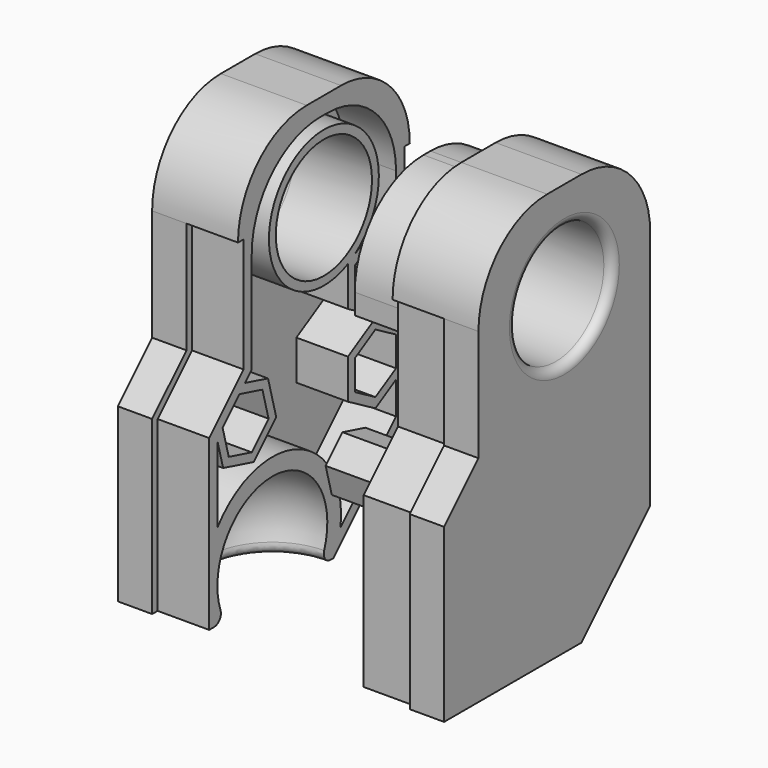
from build123d import *

# Parameters (mm, degrees)
F1_DEPTH  = 5
F4_R      = 3.5
F5_DEPTH  = 25
F7_DEPTH  = 3
F9_R      = 5
F11_DEPTH = 6
F13_DEPTH = 6
F14_R     = 0.5
F14_2_R   = 0.5
F16_DEPTH = 3
F18_DEPTH = 3


with BuildPart() as f1:
    # F0 (on Right) → F1 (new body)
    with BuildSketch(Plane.YZ):
        Polygon((0, 10), (0, 0), (10, 0), (15, 5), (15, 20), (15, 24), (2.5, 24), (2.5, 20), (2.5, 12.5), align=None)
    extrude(amount=F1_DEPTH)

    # F2 (on face) → F3 (revolve, cut)
    with BuildSketch(Plane.YZ.offset(5)):
        with BuildLine():
            Line((5, -2), (5, 6))
            ThreePointArc((5, 6), (1, 2), (5, -2))
        make_face()
    revolve(axis=Axis((5, 5, 2), (0, 0, -1)), mode=Mode.SUBTRACT)

    # F4 (on face) → F5 (cut)
    with BuildSketch(Plane.YZ.offset(5)):
        with Locations((8.75, 18.25)):
            Circle(F4_R)
    extrude(amount=-F5_DEPTH, mode=Mode.SUBTRACT)

    # F6 (on face) → F7 (cut)
    with BuildSketch(Plane.YZ.offset(5)):
        with BuildLine():
            Line((1.4182789124, 7.8827450064), (1, 9.4437831591))
            Line((1, 9.4437831591), (1, 5))
            ThreePointArc((1, 5), (6.8750834794, 6.6350902845), (9.9607833148, 1.3749968772))
            Line((9.9607833148, 1.3749968772), (14, 5.4142135624))
            Line((14, 5.4142135624), (14, 7.3028310874))
            Line((14, 7.3028310874), (12.5, 6.4368056836))
            Line((12.5, 6.4368056836), (10.5, 7.591506222))
            Line((10.5, 7.591506222), (10.5, 9.9009072988))
            Line((10.5, 9.9009072988), (12.5, 11.0556078372))
            Line((12.5, 11.0556078372), (14, 10.1895824334))
            Line((14, 10.1895824334), (14, 12.056624327))
            Line((14, 12.056624327), (12.5, 11.1905989232))
            Line((12.5, 11.1905989232), (10.5, 12.3452994616))
            Line((10.5, 12.3452994616), (10.5, 14.6531263575))
            ThreePointArc((10.5, 14.6531263575), (5.3588350084, 20.3713203436), (12.75, 18.25))
            ThreePointArc((12.75, 18.25), (12.2870669156, 16.3820712982), (11.0054211826, 14.9465055942))
            Line((11.0054211826, 14.9465055942), (12.5, 15.8094010768))
            Line((12.5, 15.8094010768), (14, 14.943375673))
            Line((14, 14.943375673), (14, 23))
            Line((14, 23), (3.5, 23))
            Line((3.5, 23), (3.5, 12.0857864376))
            Line((3.5, 12.0857864376), (3.0112326286, 11.5970190662))
            Line((3.0112326286, 11.5970190662), (4.6842652361, 11.1487313301))
            Line((4.6842652361, 11.1487313301), (5.2819822175, 8.9180211868))
            Line((5.2819822175, 8.9180211868), (3.6489890557, 7.285028025))
            Line((3.6489890557, 7.285028025), (1.4182789124, 7.8827450064))
        make_face()
        Polygon((2.6029843381, 11.1887707758), (1.3782394667, 9.9640259044), (1.8265272028, 8.2909932969), (3.4995598103, 7.8427055608), (4.7243046817, 9.0674504322), (4.2760169456, 10.7404830397), align=None)
        Polygon((12.5, 7.0141559528), (14, 7.8801813566), (14, 9.6122321642), (12.5, 10.478257568), (11, 9.6122321642), (11, 7.8801813566), align=None)
        Polygon((14, 12.6339745962), (14, 14.3660254038), (12.5, 15.2320508076), (11, 14.3660254038), (11, 12.6339745962), (12.5, 11.7679491924), align=None)
    extrude(amount=-F7_DEPTH, mode=Mode.SUBTRACT)

    # F9
    f9_edges = [f1.edges().sort_by_distance(p)[0] for p in [
        (2.5, 2.5, 24),
        (2.5, 15, 24),
        (3.5, 3.5, 23),
        (3.5, 14, 23),
    ]]
    fillet(f9_edges, radius=F9_R)


with BuildPart() as f10_1:
    # F10: instance of F1
    add(f1.part.mirror(Plane.YZ.offset(9.5)))

    # F11 (add): faces of the model
    f11_faces = [f10_1.faces().sort_by_distance(p)[0] for p in [
        (17, 12.5, 8.7462067604),
        (17, 12.5, 13.5),
        (17, 3.0512720742, 9.5157381683),
    ]]
    extrude(f11_faces, amount=F11_DEPTH)

    # F12 (on face) → F13 (join)
    with BuildSketch(Plane(origin=(17, 0, 0), x_dir=(0, -1, 0), z_dir=(-1, 0, 0))):
        with BuildLine():
            Line((-14, 18), (-14, 16.8094010768))
            Line((-14, 16.8094010768), (-12.4815780499, 16.8094010768))
            ThreePointArc((-12.4815780499, 16.8094010768), (-8.75, 22.25), (-5.0184219501, 16.8094010768))
            Line((-5.0184219501, 16.8094010768), (-3.5, 16.8094010768))
            Line((-3.5, 16.8094010768), (-3.5, 18))
            ThreePointArc((-3.5, 18), (-4.9644660941, 21.5355339059), (-8.5, 23))
            Line((-8.5, 23), (-9, 23))
            ThreePointArc((-9, 23), (-12.5355339059, 21.5355339059), (-14, 18))
        make_face()
    extrude(amount=F13_DEPTH)

    # F14#2
    f14_2_edges = [f10_1.edges().sort_by_distance(p)[0] for p in [
        (19, 5.25, 18.25),
        (17.464102, 5, 0),
    ]]
    fillet(f14_2_edges, radius=F14_2_R)

    # F17 (on face) → F18 (cut)
    with BuildSketch(Plane(origin=(14, 0, 0), x_dir=(0, -1, 0), z_dir=(-1, 0, 0))):
        Polygon((-14.6, 19), (-15, 19), (-15, 5), (-10, 0), (-9.4343145751, 0), (-14.6, 5.1656854249), align=None)
        Polygon((-0.4, 0), (0, 0), (0, 10), (-2.5, 12.5), (-2.5, 19), (-2.9, 19), (-2.9, 12.3343145751), (-0.4, 9.8343145751), align=None)
    extrude(amount=-F18_DEPTH, mode=Mode.SUBTRACT)


with BuildPart() as f1_1:
    add(f1.part)

    # F14
    f14_edges = [f1_1.edges().sort_by_distance(p)[0] for p in [
        (0, 5.25, 18.25),
        (1.535898, 5, 0),
    ]]
    fillet(f14_edges, radius=F14_R)

    # F15 (on face) → F16 (cut)
    with BuildSketch(Plane.YZ.offset(5)):
        Polygon((0, 10), (0, 0), (0.4, 0), (0.4, 9.8343145751), (2.8896803781, 12.3239949532), (2.9, 12.3343145751), (2.9, 12.8194838762), (2.9, 19), (2.5, 19), (2.5, 12.5), align=None)
        Polygon((15, 5), (15, 19), (14.6, 19), (14.6, 5.1656854249), (14.5191117842, 5.0847972091), (9.4343145751, 0), (10, 0), align=None)
    extrude(amount=-F16_DEPTH, mode=Mode.SUBTRACT)


solid = Compound([f10_1.part, f1_1.part])
